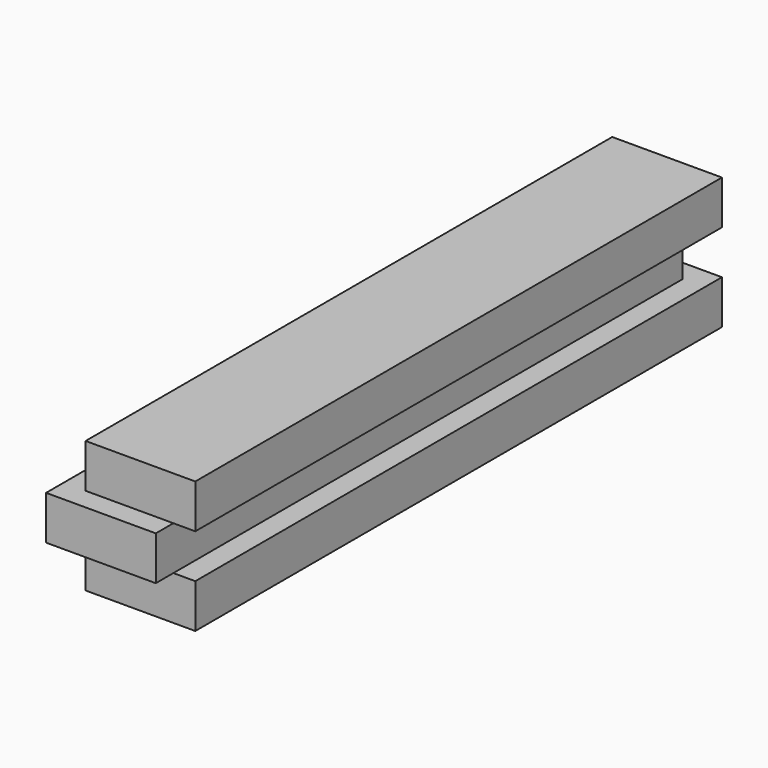
from build123d import *

# Parameters (mm, degrees)
F2_W     = 7.9375
F2_H     = 47.625
F3_DEPTH = 3.175
F4_W     = 7.9375
F4_H     = 47.625
F5_DEPTH = 3.175
F6_W     = 7.9375
F6_H     = 47.625
F7_DEPTH = 3.175


# Not quite as in the source:
# - a variable given as a bare number and used for a length is read in inches; the dataset says mm whatever the document's units were


with BuildPart() as f3:
    # F2 (on Top) → F3 (new body)
    with BuildSketch(Plane.XY):
        with Locations((3.96875, 23.8125)):
            Rectangle(F2_W, F2_H)
    extrude(amount=F3_DEPTH)

    # F4 (on face) → F5 (join)
    with BuildSketch(Plane.XY.offset(3.175)):
        with Locations((2.38125, 22.225)):
            Rectangle(F4_W, F4_H)
    extrude(amount=F5_DEPTH)

    # F6 (on face) → F7 (join)
    with BuildSketch(Plane.XY.offset(6.35)):
        with Locations((3.96875, 23.8125)):
            Rectangle(F6_W, F6_H)
    extrude(amount=F7_DEPTH)


solid = f3.part
